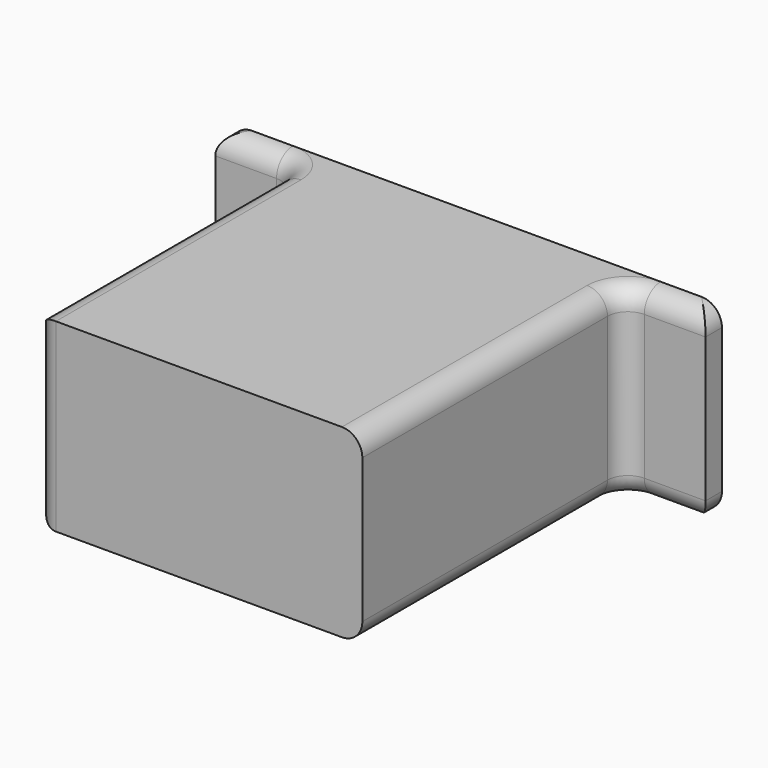
from build123d import *

# Parameters (mm, degrees)
F0_W     = 152.4
F0_H     = 57.531
F1_DEPTH = 6.35
F2_W     = 101.6
F2_H     = 57.531
F3_DEPTH = 101.6
F4_F1_R  = 6.35
F4_F2_R  = 6.3499


# Not quite as in the source:
# - a fillet or chamfer is up to 0.001 mm smaller than in the source, because OpenCascade refuses the exact size


with BuildPart() as f1:
    # F0 (on Front) → F1 (new body)
    with BuildSketch(Plane.XZ):
        Rectangle(F0_W, F0_H)
    extrude(amount=F1_DEPTH)

    # F2 (on face) → F3 (join)
    with BuildSketch(Plane.XZ.offset(6.35)):
        Rectangle(F2_W, F2_H)
    extrude(amount=F3_DEPTH)

    # F4: fillet of radius 6.35 on 11 edges, made by hand

    # F4_f1
    f4_f1_edges = [f1.edges().sort_by_distance(p)[0] for p in [
        (50.8, -6.35, 0),
        (-50.8, -6.35, 0),
    ]]
    fillet(f4_f1_edges, radius=F4_F1_R)

    # F4_f2 (radius 6.35 in the source; OpenCascade refuses exactly that, so slightly less here)
    f4_f2_edges = [f1.edges().sort_by_distance(p)[0] for p in [
        (-76.2, -3.175, -28.7655),
        (-50.8, -60.325, -28.7655),
        (-50.8, -60.325, 28.7655),
        (50.8, -60.325, -28.7655),
        (50.8, -60.325, 28.7655),
        (-50.8, -107.95, 0),
        (-76.2, -3.175, 28.7655),
        (76.2, -3.175, 28.7655),
        (76.2, -3.175, -28.7655),
        (52.6598719395, -8.2098719395, 28.7655),
        (52.6598719395, -8.2098719395, -28.7655),
        (-52.6598719395, -8.2098719395, 28.7655),
        (-52.6598719395, -8.2098719395, -28.7655),
    ]]
    fillet(f4_f2_edges, radius=F4_F2_R)


solid = f1.part
